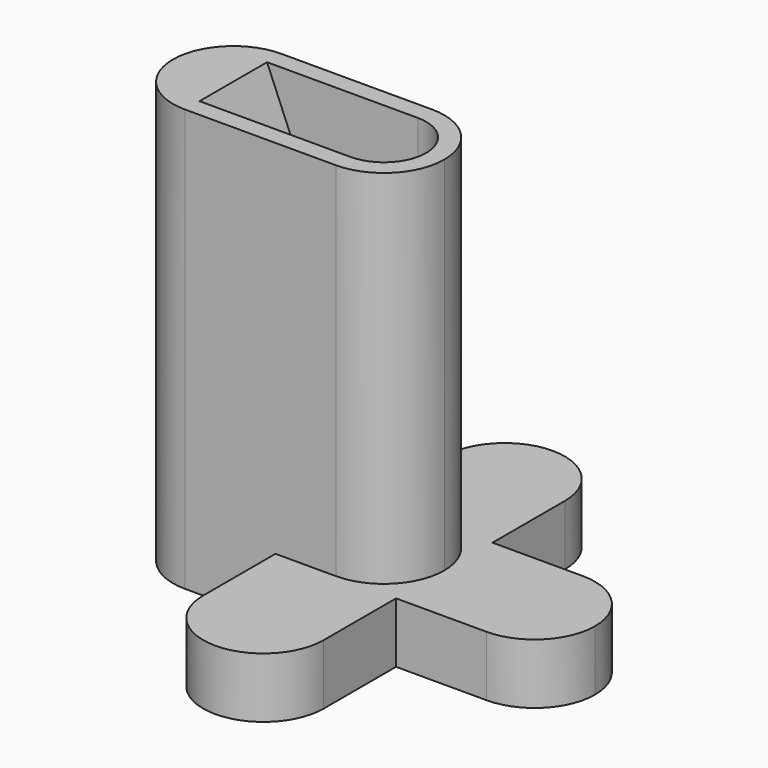
from build123d import *

# Parameters (mm, degrees)
F2_DEPTH  = 5
F3_DEPTH  = 40
F4_DEPTH  = 10
F5_DEPTH  = 40
F9_DEPTH  = 3
F10_SIZE  = 2
F12_DEPTH = 20


# Not quite as in the source:
# - a feature of the source that left no trace in its solid (it failed there, or was rolled back) is left out


with BuildPart() as f2:
    # F1 (on Front) → F2 (new body, symmetric)
    with BuildSketch(Plane.XZ):
        Polygon((-12.5, 10), (0, 10), (-12.5, 40), align=None)
    extrude(amount=F2_DEPTH, both=True)

    # F0 (on Top) → F3 (join)
    with BuildSketch(Plane.XY):
        with BuildLine():
            ThreePointArc((0, -5), (3.5355339059, -3.5355339059), (5, 0))
            ThreePointArc((5, 0), (3.5355339059, 3.5355339059), (0, 5))
            Line((0, 5), (0, 3.5))
            ThreePointArc((0, 3.5), (2.4748737342, 2.4748737342), (3.5, 0))
            ThreePointArc((3.5, 0), (2.4748737342, -2.4748737342), (0, -3.5))
            Line((0, -3.5), (0, -5))
        make_face()
        with BuildLine():
            Line((0, 3.5), (0, 5))
            ThreePointArc((0, 5), (-1.9364916731, 4.6097722286), (-3.5707142143, 3.5))
            Line((-3.5707142143, 3.5), (0, 3.5))
        make_face()
        with BuildLine():
            ThreePointArc((-3.5707142143, 3.5), (-1.9364916731, 4.6097722286), (0, 5))
            Line((0, 5), (-5, 5))
            Line((-5, 5), (-5, 3.5))
            Line((-5, 3.5), (-3.5707142143, 3.5))
        make_face()
        with BuildLine():
            Line((-5, 3.5), (-5, 5))
            Line((-5, 5), (-11.4564392374, 5))
            ThreePointArc((-11.4564392374, 5), (-11.4783307541, 4.9495376652), (-11.5, 4.8989794856))
            ThreePointArc((-11.5, 4.8989794856), (-10.1099910027, 4.3917942794), (-8.9292857857, 3.5))
            Line((-8.9292857857, 3.5), (-5, 3.5))
        make_face()
        with BuildLine():
            Line((-12, 3.5), (-8.9292857857, 3.5))
            ThreePointArc((-8.9292857857, 3.5), (-10.1099910027, 4.3917942794), (-11.5, 4.8989794856))
            ThreePointArc((-11.5, 4.8989794856), (-11.7708022624, 4.2069245417), (-12, 3.5))
        make_face()
        with BuildLine():
            ThreePointArc((-12, 3.5), (-11.7708022624, 4.2069245417), (-11.5, 4.8989794856))
            ThreePointArc((-11.5, 4.8989794856), (-11.99745519, 4.974680765), (-12.5, 5))
            Line((-12.5, 5), (-12.5, 3.5))
            Line((-12.5, 3.5), (-12, 3.5))
        make_face()
        with BuildLine():
            ThreePointArc((-12.5, -5), (-11.99745519, -4.974680765), (-11.5, -4.8989794856))
            ThreePointArc((-11.5, -4.8989794856), (-11.7708022624, -4.2069245417), (-12, -3.5))
            Line((-12, -3.5), (-12.5, -3.5))
            Line((-12.5, -3.5), (-12.5, -5))
        make_face()
        with BuildLine():
            ThreePointArc((-11.5, -4.8989794856), (-10.1099910027, -4.3917942794), (-8.9292857857, -3.5))
            Line((-8.9292857857, -3.5), (-12, -3.5))
            ThreePointArc((-12, -3.5), (-11.7708022624, -4.2069245417), (-11.5, -4.8989794856))
        make_face()
        with BuildLine():
            Line((-11.4564392374, -5), (-5, -5))
            Line((-5, -5), (-5, -3.5))
            Line((-5, -3.5), (-8.9292857857, -3.5))
            ThreePointArc((-8.9292857857, -3.5), (-10.1099910027, -4.3917942794), (-11.5, -4.8989794856))
            ThreePointArc((-11.5, -4.8989794856), (-11.4783307541, -4.9495376652), (-11.4564392374, -5))
        make_face()
        with BuildLine():
            Line((-5, -5), (0, -5))
            ThreePointArc((0, -5), (-1.9364916731, -4.6097722286), (-3.5707142143, -3.5))
            Line((-3.5707142143, -3.5), (-5, -3.5))
            Line((-5, -3.5), (-5, -5))
        make_face()
        with BuildLine():
            ThreePointArc((-3.5707142143, -3.5), (-1.9364916731, -4.6097722286), (0, -5))
            Line((0, -5), (0, -3.5))
            Line((0, -3.5), (-3.5707142143, -3.5))
        make_face()
        with BuildLine():
            Line((-12.5, -5), (-11.4564392374, -5))
            ThreePointArc((-11.4564392374, -5), (-11.4783307541, -4.9495376652), (-11.5, -4.8989794856))
            ThreePointArc((-11.5, -4.8989794856), (-11.99745519, -4.974680765), (-12.5, -5))
        make_face()
        with BuildLine():
            ThreePointArc((-11.5, 4.8989794856), (-11.4783307541, 4.9495376652), (-11.4564392374, 5))
            Line((-11.4564392374, 5), (-12.5, 5))
            ThreePointArc((-12.5, 5), (-11.99745519, 4.974680765), (-11.5, 4.8989794856))
        make_face()
        with BuildLine():
            Line((-12.5, 0), (-12.5, 3))
            ThreePointArc((-12.5, 3), (-15.5, 0), (-12.5, -3))
            Line((-12.5, -3), (-12.5, 0))
        make_face()
        with BuildLine():
            Line((-12.5, 3.5), (-12.5, 5))
            ThreePointArc((-12.5, 5), (-17.5, 0), (-12.5, -5))
            Line((-12.5, -5), (-12.5, -3.5))
            Line((-12.5, -3.5), (-12.5, -3))
            ThreePointArc((-12.5, -3), (-15.5, 0), (-12.5, 3))
            Line((-12.5, 3), (-12.5, 3.5))
        make_face()
    extrude(amount=F3_DEPTH)

    # F0 (on Top) → F5 (cut)
    with BuildSketch(Plane.XY):
        with BuildLine():
            ThreePointArc((3.5, 0), (2.4748737342, 2.4748737342), (0, 3.5))
            ThreePointArc((0, 3.5), (-3.5, 0), (0, -3.5))
            ThreePointArc((0, -3.5), (2.4748737342, -2.4748737342), (3.5, 0))
        make_face()
    extrude(amount=F5_DEPTH, mode=Mode.SUBTRACT)


with BuildPart() as f4:
    # F0 (on Top) → F4 (new body)
    with BuildSketch(Plane.XY):
        with BuildLine():
            Line((0, 3.5), (-3.5707142143, 3.5))
            ThreePointArc((-3.5707142143, 3.5), (-4.6289075964, 1.8902948088), (-5, 0))
            ThreePointArc((-5, 0), (-4.6289075964, -1.8902948088), (-3.5707142143, -3.5))
            Line((-3.5707142143, -3.5), (0, -3.5))
            ThreePointArc((0, -3.5), (-3.5, 0), (0, 3.5))
        make_face()
        with BuildLine():
            ThreePointArc((-5, 0), (-4.6289075964, 1.8902948088), (-3.5707142143, 3.5))
            Line((-3.5707142143, 3.5), (-5, 3.5))
            Line((-5, 3.5), (-5, 0))
        make_face()
        with BuildLine():
            Line((-5, -3.5), (-3.5707142143, -3.5))
            ThreePointArc((-3.5707142143, -3.5), (-4.6289075964, -1.8902948088), (-5, 0))
            Line((-5, 0), (-5, -3.5))
        make_face()
        with BuildLine():
            Line((-5, -3.5), (-5, 0))
            Line((-5, 0), (-5, 3.5))
            Line((-5, 3.5), (-8.9292857857, 3.5))
            ThreePointArc((-8.9292857857, 3.5), (-7.8710924036, 1.8902948088), (-7.5, 0))
            ThreePointArc((-7.5, 0), (-7.8710924036, -1.8902948088), (-8.9292857857, -3.5))
            Line((-8.9292857857, -3.5), (-5, -3.5))
        make_face()
        with BuildLine():
            ThreePointArc((-7.5, 0), (-7.8710924036, 1.8902948088), (-8.9292857857, 3.5))
            Line((-8.9292857857, 3.5), (-12, 3.5))
            ThreePointArc((-12, 3.5), (-12.072818108, 3.239917118), (-12.14, 2.978321675))
            ThreePointArc((-12.14, 2.978321675), (-10.2550055679, 1.9899748742), (-9.5, 0))
            ThreePointArc((-9.5, 0), (-10.2550055679, -1.9899748742), (-12.14, -2.978321675))
            ThreePointArc((-12.14, -2.978321675), (-12.072818108, -3.239917118), (-12, -3.5))
            Line((-12, -3.5), (-8.9292857857, -3.5))
            ThreePointArc((-8.9292857857, -3.5), (-7.8710924036, -1.8902948088), (-7.5, 0))
        make_face()
        with BuildLine():
            ThreePointArc((-9.5, 0), (-10.2550055679, 1.9899748742), (-12.14, 2.978321675))
            ThreePointArc((-12.14, 2.978321675), (-12.409673646, 1.5), (-12.5, 0))
            ThreePointArc((-12.5, 0), (-12.409673646, -1.5), (-12.14, -2.978321675))
            ThreePointArc((-12.14, -2.978321675), (-10.2550055679, -1.9899748742), (-9.5, 0))
        make_face()
        with BuildLine():
            ThreePointArc((-12.5, 0), (-12.409673646, 1.5), (-12.14, 2.978321675))
            ThreePointArc((-12.14, 2.978321675), (-12.3196739413, 2.9945755146), (-12.5, 3))
            Line((-12.5, 3), (-12.5, 0))
        make_face()
        with BuildLine():
            ThreePointArc((-12.5, -3), (-12.3196739413, -2.9945755146), (-12.14, -2.978321675))
            ThreePointArc((-12.14, -2.978321675), (-12.409673646, -1.5), (-12.5, 0))
            Line((-12.5, 0), (-12.5, -3))
        make_face()
        with BuildLine():
            Line((-12.5, -3.5), (-12, -3.5))
            ThreePointArc((-12, -3.5), (-12.072818108, -3.239917118), (-12.14, -2.978321675))
            ThreePointArc((-12.14, -2.978321675), (-12.3196739413, -2.9945755146), (-12.5, -3))
            Line((-12.5, -3), (-12.5, -3.5))
        make_face()
        with BuildLine():
            ThreePointArc((-12.14, 2.978321675), (-12.072818108, 3.239917118), (-12, 3.5))
            Line((-12, 3.5), (-12.5, 3.5))
            Line((-12.5, 3.5), (-12.5, 3))
            ThreePointArc((-12.5, 3), (-12.3196739413, 2.9945755146), (-12.14, 2.978321675))
        make_face()
    extrude(amount=F4_DEPTH)


with BuildPart() as f4b:
    # F0 (on Top) → F4, piece 2 (new body)
    with BuildSketch(Plane.XY):
        with BuildLine():
            Line((5, 5), (5, 11.4564392374))
            ThreePointArc((5, 11.4564392374), (4.9495376652, 11.4783307541), (4.8989794856, 11.5))
            ThreePointArc((4.8989794856, 11.5), (0, 7.5), (-4.8989794856, 11.5))
            ThreePointArc((-4.8989794856, 11.5), (-4.9495376652, 11.4783307541), (-5, 11.4564392374))
            Line((-5, 11.4564392374), (-5, 5))
            Line((-5, 5), (0, 5))
            Line((0, 5), (5, 5))
        make_face()
        with BuildLine():
            ThreePointArc((-4.8989794856, 11.5), (0, 7.5), (4.8989794856, 11.5))
            ThreePointArc((4.8989794856, 11.5), (3.9516285749, 11.8589473229), (2.978321675, 12.14))
            ThreePointArc((2.978321675, 12.14), (0, 9.5), (-2.978321675, 12.14))
            ThreePointArc((-2.978321675, 12.14), (-3.9516285749, 11.8589473229), (-4.8989794856, 11.5))
        make_face()
        with BuildLine():
            ThreePointArc((-2.978321675, 12.14), (0, 9.5), (2.978321675, 12.14))
            ThreePointArc((2.978321675, 12.14), (1.5, 12.409673646), (0, 12.5))
            ThreePointArc((0, 12.5), (-1.5, 12.409673646), (-2.978321675, 12.14))
        make_face()
        with BuildLine():
            ThreePointArc((0, 12.5), (1.5, 12.409673646), (2.978321675, 12.14))
            ThreePointArc((2.978321675, 12.14), (2.9945755146, 12.3196739413), (3, 12.5))
            Line((3, 12.5), (0, 12.5))
        make_face()
        with BuildLine():
            ThreePointArc((2.978321675, 12.14), (3.9516285749, 11.8589473229), (4.8989794856, 11.5))
            ThreePointArc((4.8989794856, 11.5), (4.974680765, 11.99745519), (5, 12.5))
            Line((5, 12.5), (3, 12.5))
            ThreePointArc((3, 12.5), (2.9945755146, 12.3196739413), (2.978321675, 12.14))
        make_face()
        with BuildLine():
            Line((3, 12.5), (5, 12.5))
            ThreePointArc((5, 12.5), (0, 17.5), (-5, 12.5))
            Line((-5, 12.5), (-3, 12.5))
            ThreePointArc((-3, 12.5), (0, 15.5), (3, 12.5))
        make_face()
        with BuildLine():
            Line((0, 12.5), (3, 12.5))
            ThreePointArc((3, 12.5), (0, 15.5), (-3, 12.5))
            Line((-3, 12.5), (0, 12.5))
        make_face()
        with BuildLine():
            ThreePointArc((-2.978321675, 12.14), (-1.5, 12.409673646), (0, 12.5))
            Line((0, 12.5), (-3, 12.5))
            ThreePointArc((-3, 12.5), (-2.9945755146, 12.3196739413), (-2.978321675, 12.14))
        make_face()
        with BuildLine():
            ThreePointArc((-5, 12.5), (-4.974680765, 11.99745519), (-4.8989794856, 11.5))
            ThreePointArc((-4.8989794856, 11.5), (-3.9516285749, 11.8589473229), (-2.978321675, 12.14))
            ThreePointArc((-2.978321675, 12.14), (-2.9945755146, 12.3196739413), (-3, 12.5))
            Line((-3, 12.5), (-5, 12.5))
        make_face()
        with BuildLine():
            ThreePointArc((12.14, -2.978321675), (9.5, 0), (12.14, 2.978321675))
            ThreePointArc((12.14, 2.978321675), (11.8589473229, 3.9516285749), (11.5, 4.8989794856))
            ThreePointArc((11.5, 4.8989794856), (7.5, 0), (11.5, -4.8989794856))
            ThreePointArc((11.5, -4.8989794856), (11.8589473229, -3.9516285749), (12.14, -2.978321675))
        make_face()
        with BuildLine():
            ThreePointArc((11.5, 4.8989794856), (11.8589473229, 3.9516285749), (12.14, 2.978321675))
            ThreePointArc((12.14, 2.978321675), (12.3196739413, 2.9945755146), (12.5, 3))
            Line((12.5, 3), (12.5, 5))
            ThreePointArc((12.5, 5), (11.99745519, 4.974680765), (11.5, 4.8989794856))
        make_face()
        with BuildLine():
            Line((12.5, 5), (12.5, 3))
            ThreePointArc((12.5, 3), (14.6213203436, 2.1213203436), (15.5, 0))
            ThreePointArc((15.5, 0), (14.6213203436, -2.1213203436), (12.5, -3))
            Line((12.5, -3), (12.5, -5))
            ThreePointArc((12.5, -5), (16.0355339059, -3.5355339059), (17.5, 0))
            ThreePointArc((17.5, 0), (16.0355339059, 3.5355339059), (12.5, 5))
        make_face()
        with BuildLine():
            Line((12.5, 3), (12.5, 0))
            Line((12.5, 0), (12.5, -3))
            ThreePointArc((12.5, -3), (14.6213203436, -2.1213203436), (15.5, 0))
            ThreePointArc((15.5, 0), (14.6213203436, 2.1213203436), (12.5, 3))
        make_face()
        with BuildLine():
            ThreePointArc((12.14, -2.978321675), (12.409673646, -1.5), (12.5, 0))
            ThreePointArc((12.5, 0), (12.409673646, 1.5), (12.14, 2.978321675))
            ThreePointArc((12.14, 2.978321675), (9.5, 0), (12.14, -2.978321675))
        make_face()
        with BuildLine():
            ThreePointArc((12.14, 2.978321675), (12.409673646, 1.5), (12.5, 0))
            Line((12.5, 0), (12.5, 3))
            ThreePointArc((12.5, 3), (12.3196739413, 2.9945755146), (12.14, 2.978321675))
        make_face()
        with BuildLine():
            Line((12.5, -3), (12.5, 0))
            ThreePointArc((12.5, 0), (12.409673646, -1.5), (12.14, -2.978321675))
            ThreePointArc((12.14, -2.978321675), (12.3196739413, -2.9945755146), (12.5, -3))
        make_face()
        with BuildLine():
            ThreePointArc((12.5, -3), (12.3196739413, -2.9945755146), (12.14, -2.978321675))
            ThreePointArc((12.14, -2.978321675), (11.8589473229, -3.9516285749), (11.5, -4.8989794856))
            ThreePointArc((11.5, -4.8989794856), (11.99745519, -4.974680765), (12.5, -5))
            Line((12.5, -5), (12.5, -3))
        make_face()
        with BuildLine():
            ThreePointArc((11.5, -4.8989794856), (7.5, 0), (11.5, 4.8989794856))
            ThreePointArc((11.5, 4.8989794856), (11.4783307541, 4.9495376652), (11.4564392374, 5))
            Line((11.4564392374, 5), (5, 5))
            Line((5, 5), (5, 0))
            Line((5, 0), (5, -5))
            Line((5, -5), (11.4564392374, -5))
            ThreePointArc((11.4564392374, -5), (11.4783307541, -4.9495376652), (11.5, -4.8989794856))
        make_face()
        with BuildLine():
            ThreePointArc((4.8989794856, 11.5), (4.9495376652, 11.4783307541), (5, 11.4564392374))
            Line((5, 11.4564392374), (5, 12.5))
            ThreePointArc((5, 12.5), (4.974680765, 11.99745519), (4.8989794856, 11.5))
        make_face()
        with BuildLine():
            ThreePointArc((-5, 11.4564392374), (-4.9495376652, 11.4783307541), (-4.8989794856, 11.5))
            ThreePointArc((-4.8989794856, 11.5), (-4.974680765, 11.99745519), (-5, 12.5))
            Line((-5, 12.5), (-5, 11.4564392374))
        make_face()
        with BuildLine():
            ThreePointArc((11.4564392374, 5), (11.4783307541, 4.9495376652), (11.5, 4.8989794856))
            ThreePointArc((11.5, 4.8989794856), (11.99745519, 4.974680765), (12.5, 5))
            Line((12.5, 5), (11.4564392374, 5))
        make_face()
        with BuildLine():
            ThreePointArc((12.5, -5), (11.99745519, -4.974680765), (11.5, -4.8989794856))
            ThreePointArc((11.5, -4.8989794856), (11.4783307541, -4.9495376652), (11.4564392374, -5))
            Line((11.4564392374, -5), (12.5, -5))
        make_face()
        with BuildLine():
            ThreePointArc((-5, -12.5), (0, -17.5), (5, -12.5))
            Line((5, -12.5), (3, -12.5))
            ThreePointArc((3, -12.5), (0, -15.5), (-3, -12.5))
            Line((-3, -12.5), (-5, -12.5))
        make_face()
        with BuildLine():
            ThreePointArc((3, -12.5), (2.9945755146, -12.3196739413), (2.978321675, -12.14))
            ThreePointArc((2.978321675, -12.14), (1.5, -12.409673646), (0, -12.5))
            Line((0, -12.5), (3, -12.5))
        make_face()
        with BuildLine():
            ThreePointArc((5, -12.5), (4.974680765, -11.99745519), (4.8989794856, -11.5))
            ThreePointArc((4.8989794856, -11.5), (3.9516285749, -11.8589473229), (2.978321675, -12.14))
            ThreePointArc((2.978321675, -12.14), (2.9945755146, -12.3196739413), (3, -12.5))
            Line((3, -12.5), (5, -12.5))
        make_face()
        with BuildLine():
            ThreePointArc((-3, -12.5), (0, -15.5), (3, -12.5))
            Line((3, -12.5), (0, -12.5))
            Line((0, -12.5), (-3, -12.5))
        make_face()
        with BuildLine():
            ThreePointArc((0, -12.5), (1.5, -12.409673646), (2.978321675, -12.14))
            ThreePointArc((2.978321675, -12.14), (0, -9.5), (-2.978321675, -12.14))
            ThreePointArc((-2.978321675, -12.14), (-1.5, -12.409673646), (0, -12.5))
        make_face()
        with BuildLine():
            ThreePointArc((2.978321675, -12.14), (3.9516285749, -11.8589473229), (4.8989794856, -11.5))
            ThreePointArc((4.8989794856, -11.5), (0, -7.5), (-4.8989794856, -11.5))
            ThreePointArc((-4.8989794856, -11.5), (-3.9516285749, -11.8589473229), (-2.978321675, -12.14))
            ThreePointArc((-2.978321675, -12.14), (0, -9.5), (2.978321675, -12.14))
        make_face()
        with BuildLine():
            ThreePointArc((-2.978321675, -12.14), (-3.9516285749, -11.8589473229), (-4.8989794856, -11.5))
            ThreePointArc((-4.8989794856, -11.5), (-4.974680765, -11.99745519), (-5, -12.5))
            Line((-5, -12.5), (-3, -12.5))
            ThreePointArc((-3, -12.5), (-2.9945755146, -12.3196739413), (-2.978321675, -12.14))
        make_face()
        with BuildLine():
            Line((-3, -12.5), (0, -12.5))
            ThreePointArc((0, -12.5), (-1.5, -12.409673646), (-2.978321675, -12.14))
            ThreePointArc((-2.978321675, -12.14), (-2.9945755146, -12.3196739413), (-3, -12.5))
        make_face()
        with BuildLine():
            ThreePointArc((4.8989794856, -11.5), (4.9495376652, -11.4783307541), (5, -11.4564392374))
            Line((5, -11.4564392374), (5, -5))
            Line((5, -5), (0, -5))
            Line((0, -5), (-5, -5))
            Line((-5, -5), (-5, -11.4564392374))
            ThreePointArc((-5, -11.4564392374), (-4.9495376652, -11.4783307541), (-4.8989794856, -11.5))
            ThreePointArc((-4.8989794856, -11.5), (0, -7.5), (4.8989794856, -11.5))
        make_face()
        with BuildLine():
            Line((5, -12.5), (5, -11.4564392374))
            ThreePointArc((5, -11.4564392374), (4.9495376652, -11.4783307541), (4.8989794856, -11.5))
            ThreePointArc((4.8989794856, -11.5), (4.974680765, -11.99745519), (5, -12.5))
        make_face()
        with BuildLine():
            ThreePointArc((-5, -12.5), (-4.974680765, -11.99745519), (-4.8989794856, -11.5))
            ThreePointArc((-4.8989794856, -11.5), (-4.9495376652, -11.4783307541), (-5, -11.4564392374))
            Line((-5, -11.4564392374), (-5, -12.5))
        make_face()
        with BuildLine():
            Line((5, 0), (5, 5))
            Line((5, 5), (0, 5))
            ThreePointArc((0, 5), (3.5355339059, 3.5355339059), (5, 0))
        make_face()
        with BuildLine():
            Line((0, -5), (5, -5))
            Line((5, -5), (5, 0))
            ThreePointArc((5, 0), (3.5355339059, -3.5355339059), (0, -5))
        make_face()
    extrude(amount=F4_DEPTH)

    # F0 (on Top) → F9 (join)
    with BuildSketch(Plane.XY):
        with BuildLine():
            Line((12.5, -3), (12.5, 0))
            ThreePointArc((12.5, 0), (12.409673646, -1.5), (12.14, -2.978321675))
            ThreePointArc((12.14, -2.978321675), (12.3196739413, -2.9945755146), (12.5, -3))
        make_face()
        with BuildLine():
            ThreePointArc((12.14, -2.978321675), (12.409673646, -1.5), (12.5, 0))
            ThreePointArc((12.5, 0), (12.409673646, 1.5), (12.14, 2.978321675))
            ThreePointArc((12.14, 2.978321675), (9.5, 0), (12.14, -2.978321675))
        make_face()
        with BuildLine():
            ThreePointArc((12.14, 2.978321675), (12.409673646, 1.5), (12.5, 0))
            Line((12.5, 0), (12.5, 3))
            ThreePointArc((12.5, 3), (12.3196739413, 2.9945755146), (12.14, 2.978321675))
        make_face()
        with BuildLine():
            Line((12.5, 3), (12.5, 0))
            Line((12.5, 0), (12.5, -3))
            ThreePointArc((12.5, -3), (14.6213203436, -2.1213203436), (15.5, 0))
            ThreePointArc((15.5, 0), (14.6213203436, 2.1213203436), (12.5, 3))
        make_face()
        with BuildLine():
            ThreePointArc((-3, -12.5), (0, -15.5), (3, -12.5))
            Line((3, -12.5), (0, -12.5))
            Line((0, -12.5), (-3, -12.5))
        make_face()
        with BuildLine():
            ThreePointArc((0, -12.5), (1.5, -12.409673646), (2.978321675, -12.14))
            ThreePointArc((2.978321675, -12.14), (0, -9.5), (-2.978321675, -12.14))
            ThreePointArc((-2.978321675, -12.14), (-1.5, -12.409673646), (0, -12.5))
        make_face()
        with BuildLine():
            ThreePointArc((3, -12.5), (2.9945755146, -12.3196739413), (2.978321675, -12.14))
            ThreePointArc((2.978321675, -12.14), (1.5, -12.409673646), (0, -12.5))
            Line((0, -12.5), (3, -12.5))
        make_face()
        with BuildLine():
            Line((-3, -12.5), (0, -12.5))
            ThreePointArc((0, -12.5), (-1.5, -12.409673646), (-2.978321675, -12.14))
            ThreePointArc((-2.978321675, -12.14), (-2.9945755146, -12.3196739413), (-3, -12.5))
        make_face()
    extrude(amount=-F9_DEPTH)

    # F10
    f10_edges = [f4b.edges().sort_by_distance(p)[0] for p in [
        (2.978322, -12.86, -3),
        (12.5, 3, -3),
    ]]
    chamfer(f10_edges, length=F10_SIZE)


with BuildPart() as f12_tool:
    # F11 (on Front) → F12 (new body, symmetric)
    with BuildSketch(Plane.XZ):
        Polygon((19.8633912951, 45), (-19.8633912951, 45), (-19.8633912951, 5), (0, 5), (19.8633912951, 5), align=None)
    extrude(amount=F12_DEPTH, both=True)


with BuildPart() as f2_1:
    add(f2.part)

    # F12: intersect by f12_tool
    add(f12_tool.part, mode=Mode.INTERSECT)


with BuildPart() as f4_1:
    add(f4.part)

    # F12: intersect by f12_tool
    add(f12_tool.part, mode=Mode.INTERSECT)


with BuildPart() as f4b_1:
    add(f4b.part)

    # F12: intersect by f12_tool
    add(f12_tool.part, mode=Mode.INTERSECT)


solid = Compound([f2_1.part, f4_1.part, f4b_1.part])
